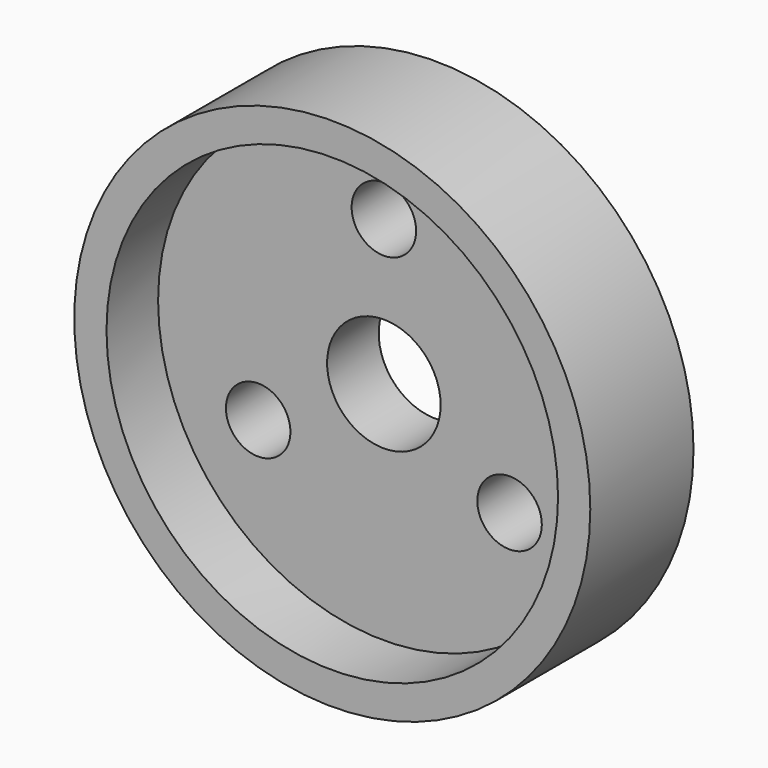
from build123d import *

# Parameters (mm, degrees)
F0_R     = 50.8
F0_R_2   = 44.45
F0_R_3   = 11.176
F1_DEPTH = 12.7
F2_R     = 6.35
F2_R_2   = 11.176
F3_DEPTH = 12.701
F2_R_3   = 50.8
F2_R_4   = 44.45
F4_DEPTH = 12.7


# Not quite as in the source:
# - a feature names something its author has since deleted; it is built from what else it names


with BuildPart() as f1:
    # F0 (on Front) → F1 (new body)
    with BuildSketch(Plane.XZ):
        Circle(F0_R)
        Circle(F0_R_2, mode=Mode.SUBTRACT)
        Circle(F0_R_2)
        Circle(F0_R_3, mode=Mode.SUBTRACT)
        Circle(F0_R_3)
    extrude(amount=F1_DEPTH)

    # F2 (on face) → F3 (cut, through all)
    with BuildSketch(Plane.XZ.offset(12.7)):
        with Locations((0, 28.575)):
            Circle(F2_R)
        with Locations((-24.7466759131, -14.2875)):
            Circle(F2_R)
        Circle(F2_R_2)
        with Locations((24.7466759131, -14.2875)):
            Circle(F2_R)
    extrude(amount=-F3_DEPTH, mode=Mode.SUBTRACT)

    # F2 (on face) → F4 (join)
    with BuildSketch(Plane.XZ.offset(12.7)):
        Circle(F2_R_3)
        Circle(F2_R_4, mode=Mode.SUBTRACT)
    extrude(amount=F4_DEPTH)


solid = f1.part
